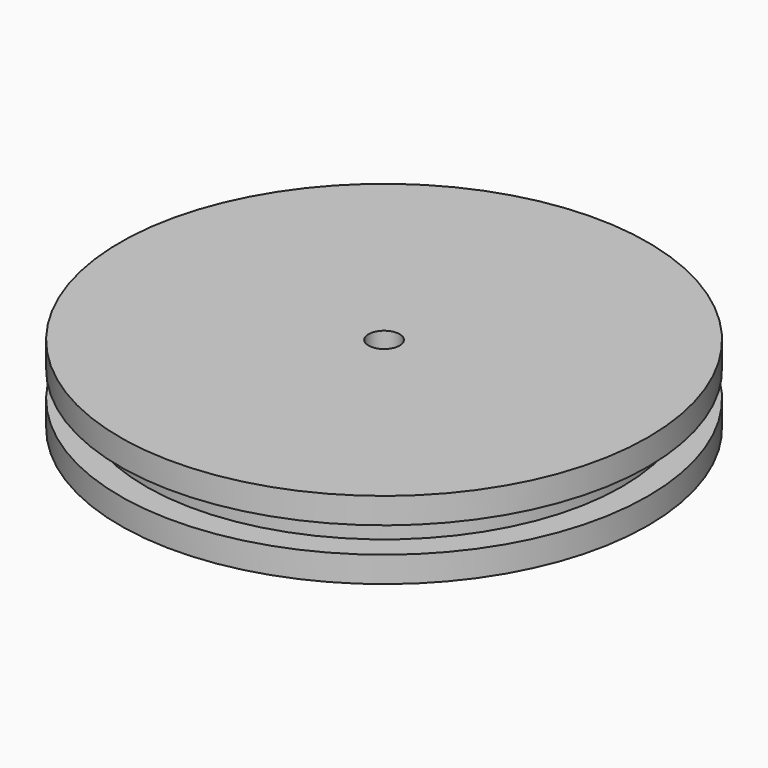
from build123d import *

# Parameters (mm, degrees)
F0_R     = 58.42
F1_DEPTH = 6.35
F2_R     = 3.81
F3_DEPTH = 25.4
F4_R     = 64.77
F4_R_2   = 58.42
F4_R_3   = 3.81
F5_DEPTH = 6.35
F6_R     = 64.77
F6_R_2   = 58.42
F6_R_3   = 3.81
F7_DEPTH = 6.35


with BuildPart() as f1:
    # F0 (on Top) → F1 (new body)
    with BuildSketch(Plane.XY):
        Circle(F0_R)
    extrude(amount=F1_DEPTH)

    # F2 (on face) → F3 (cut)
    with BuildSketch(Plane.XY.offset(6.35)):
        Circle(F2_R)
    extrude(amount=-F3_DEPTH, mode=Mode.SUBTRACT)

    # F4 (on face) → F5 (join)
    with BuildSketch(Plane.XY.offset(6.35)):
        Circle(F4_R)
        Circle(F4_R_2, mode=Mode.SUBTRACT)
        Circle(F4_R_2)
        Circle(F4_R_3, mode=Mode.SUBTRACT)
    extrude(amount=F5_DEPTH)

    # F6 (on face) → F7 (join)
    with BuildSketch(Plane(origin=(0, 0, 0), x_dir=(1, 0, 0), z_dir=(0, 0, -1))):
        Circle(F6_R)
        Circle(F6_R_2, mode=Mode.SUBTRACT)
        Circle(F6_R_2)
        Circle(F6_R_3, mode=Mode.SUBTRACT)
    extrude(amount=F7_DEPTH)


solid = f1.part
